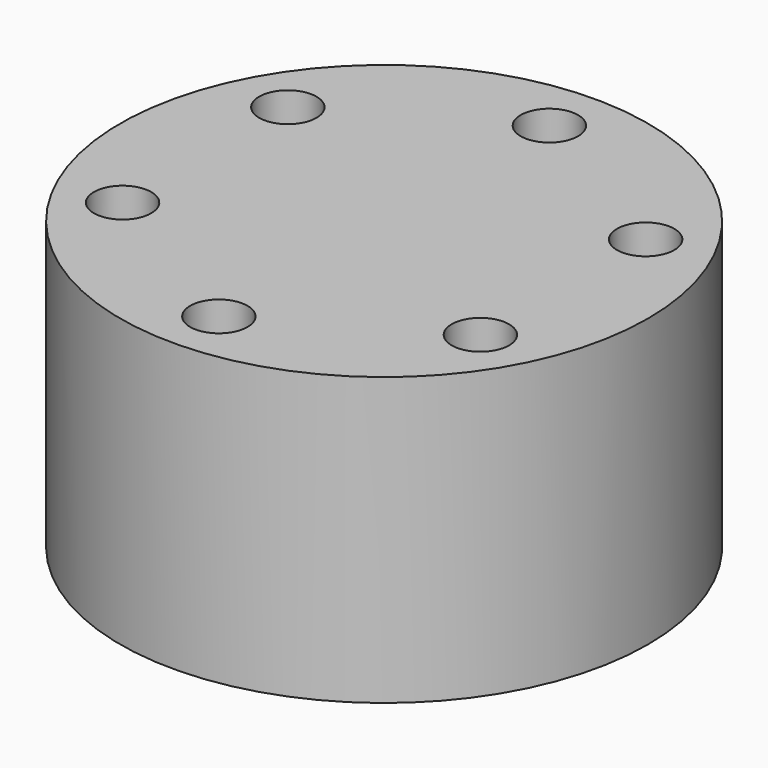
from build123d import *

# Parameters (mm, degrees)
F0_R     = 23
F4_DEPTH = 25
F6_R     = 2.5
F1_DEPTH = 15
F2_DEPTH = 4
F8_R     = 1.5
F3_DEPTH = 35


# Not quite as in the source:
# - a feature names something its author has since deleted; it is built from what else it names


with BuildPart() as f4:
    # F0 (on Top) → F4 (new body)
    with BuildSketch(Plane.XY):
        Circle(F0_R)
        with BuildLine():
            ThreePointArc((4.85, 3.616628264), (5.7421685799, 1.9052558883), (6.05, 0))
            ThreePointArc((6.05, 0), (5.7421685799, -1.9052558883), (4.85, -3.616628264))
            Line((4.85, -3.616628264), (4.85, -4.85))
            Line((4.85, -4.85), (3.616628264, -4.85))
            ThreePointArc((3.616628264, -4.85), (0, -6.05), (-3.616628264, -4.85))
            Line((-3.616628264, -4.85), (-4.85, -4.85))
            Line((-4.85, -4.85), (-4.85, -3.616628264))
            ThreePointArc((-4.85, -3.616628264), (-6.05, 0), (-4.85, 3.616628264))
            Line((-4.85, 3.616628264), (-4.85, 4.85))
            Line((-4.85, 4.85), (-3.616628264, 4.85))
            ThreePointArc((-3.616628264, 4.85), (0, 6.05), (3.616628264, 4.85))
            Line((3.616628264, 4.85), (4.85, 4.85))
            Line((4.85, 4.85), (4.85, 3.616628264))
        make_face(mode=Mode.SUBTRACT)
        with BuildLine():
            ThreePointArc((3.616628264, 4.85), (4.2779960262, 4.2779960262), (4.85, 3.616628264))
            Line((4.85, 3.616628264), (4.85, 4.85))
            Line((4.85, 4.85), (3.616628264, 4.85))
        make_face()
        with BuildLine():
            Line((-3.616628264, 4.85), (3.616628264, 4.85))
            ThreePointArc((3.616628264, 4.85), (0, 6.05), (-3.616628264, 4.85))
        make_face()
        with BuildLine():
            ThreePointArc((-4.85, 3.616628264), (-4.2779960262, 4.2779960262), (-3.616628264, 4.85))
            Line((-3.616628264, 4.85), (-4.85, 4.85))
            Line((-4.85, 4.85), (-4.85, 3.616628264))
        make_face()
        with BuildLine():
            Line((-4.85, -4.85), (-3.616628264, -4.85))
            ThreePointArc((-3.616628264, -4.85), (-4.2779960262, -4.2779960262), (-4.85, -3.616628264))
            Line((-4.85, -3.616628264), (-4.85, -4.85))
        make_face()
        with BuildLine():
            Line((4.85, -4.85), (4.85, -3.616628264))
            ThreePointArc((4.85, -3.616628264), (4.2779960262, -4.2779960262), (3.616628264, -4.85))
            Line((3.616628264, -4.85), (4.85, -4.85))
        make_face()
    extrude(amount=F4_DEPTH)

    # F6 (on face) → F1 (cut)
    with BuildSketch(Plane.XY.offset(25)):
        with Locations((15.5884572681, 9)):
            Circle(F6_R)
        with Locations((0, 18)):
            Circle(F6_R)
        with Locations((-15.5884572681, 9)):
            Circle(F6_R)
        with Locations((15.5884572681, -9)):
            Circle(F6_R)
        with Locations((0, -18)):
            Circle(F6_R)
        with Locations((-15.5884572681, -9)):
            Circle(F6_R)
    extrude(amount=-F1_DEPTH, mode=Mode.SUBTRACT)

    # F7 (on face) → F2 (join)
    with BuildSketch(Plane.XY.offset(25)):
        with BuildLine():
            Line((3.616628264, 4.85), (-3.616628264, 4.85))
            ThreePointArc((-3.616628264, 4.85), (0, -6.05), (3.616628264, 4.85))
        make_face()
    extrude(amount=-F2_DEPTH)

    # F8 (on face) → F3 (cut)
    with BuildSketch(Plane.XZ.offset(-4.85)):
        with Locations((0, 10.5)):
            Circle(F8_R)
    extrude(amount=-F3_DEPTH, mode=Mode.SUBTRACT)


solid = f4.part
